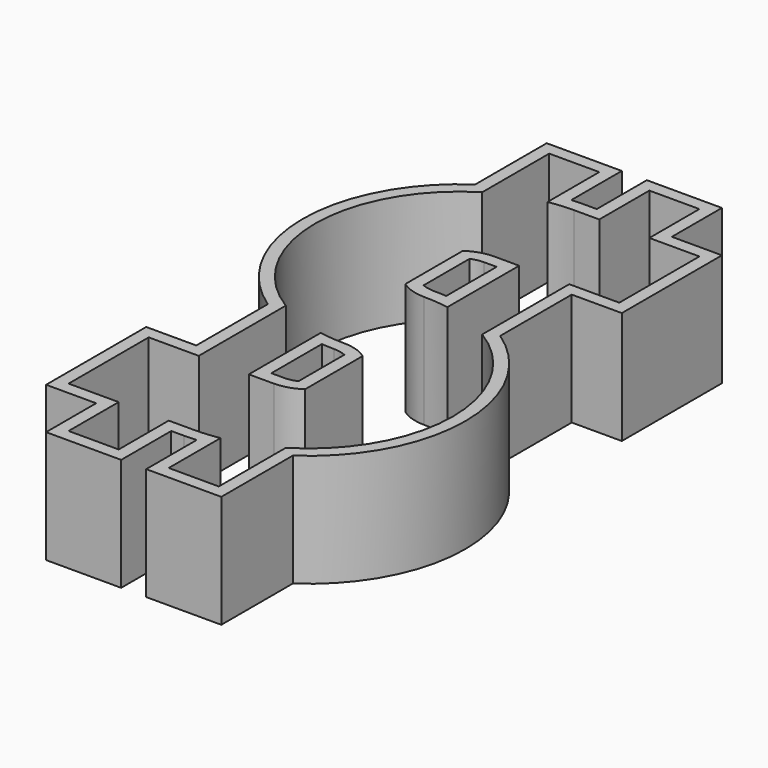
from build123d import *

# Parameters (mm, degrees)
F2_W     = 25.4
F2_H     = 25.4
F4_W     = 15.24
F4_H     = 12.7
F5_DEPTH = 25.4
F6_T     = -2.54
F7_DEPTH = 2.54


with BuildPart() as f3:
    # F3: sweep along a path in F0
    with BuildLine(Plane.XY) as f3_path:
        Line((27.94, 38.1), (0, 38.1))
        ThreePointArc((0, 38.1), (-19.05, 19.05), (0, 0))
        ThreePointArc((0, 0), (19.05, -19.05), (0, -38.1))
        Line((0, -38.1), (-27.94, -38.1))
    # F2 (on offset) → F3 (sweep)
    with BuildSketch(Plane.YZ.offset(27.94)):
        with Locations((38.1, 0)):
            Rectangle(F2_W, F2_H)
    sweep(path=f3_path.line)

    # F4 (on face) → F5 (join)
    with BuildSketch(Plane.XY.offset(12.7)):
        with BuildLine():
            Line((-2.54, 63.5), (-17.78, 63.5))
            Line((-17.78, 63.5), (-17.78, 45.3546402751))
            ThreePointArc((-17.78, 45.3546402751), (-10.5054322267, 49.0116153391), (-2.54, 50.6982369177))
            Line((-2.54, 50.6982369177), (-2.54, 63.5))
        make_face()
        with BuildLine():
            ThreePointArc((-2.54, 50.6982369177), (-10.5054322267, 49.0116153391), (-17.78, 45.3546402751))
            Line((-17.78, 45.3546402751), (-17.78, -7.2546402751))
            ThreePointArc((-17.78, -7.2546402751), (-10.5054322267, -10.9116153391), (-2.54, -12.5982369177))
            Line((-2.54, -12.5982369177), (-2.54, 13.2301288674))
            ThreePointArc((-2.54, 13.2301288674), (-6.35, 19.05), (-2.54, 24.8698711326))
            Line((-2.54, 24.8698711326), (-2.54, 50.6982369177))
        make_face()
        with BuildLine():
            ThreePointArc((-2.54, -12.5982369177), (-10.5054322267, -10.9116153391), (-17.78, -7.2546402751))
            Line((-17.78, -7.2546402751), (-17.78, -25.4))
            Line((-17.78, -25.4), (-2.54, -25.4))
            Line((-2.54, -25.4), (-2.54, -12.5982369177))
        make_face()
        with BuildLine():
            Line((-2.54, 13.2301288674), (-2.54, 24.8698711326))
            ThreePointArc((-2.54, 24.8698711326), (-6.35, 19.05), (-2.54, 13.2301288674))
        make_face()
        with Locations((10.16, 57.15)):
            Rectangle(F4_W, F4_H)
        with Locations((-10.16, -57.15)):
            Rectangle(F4_W, F4_H)
        with BuildLine():
            Line((17.78, 25.4), (2.54, 25.4))
            Line((2.54, 25.4), (2.54, 12.5982369177))
            ThreePointArc((2.54, 12.5982369177), (10.5054322267, 10.9116153391), (17.78, 7.2546402751))
            Line((17.78, 7.2546402751), (17.78, 25.4))
        make_face()
        with BuildLine():
            ThreePointArc((2.54, -24.8698711326), (6.35, -19.05), (2.54, -13.2301288674))
            Line((2.54, -13.2301288674), (2.54, -24.8698711326))
        make_face()
        with BuildLine():
            ThreePointArc((17.78, -45.3546402751), (10.5054322267, -49.0116153391), (2.54, -50.6982369177))
            Line((2.54, -50.6982369177), (2.54, -63.5))
            Line((2.54, -63.5), (17.78, -63.5))
            Line((17.78, -63.5), (17.78, -45.3546402751))
        make_face()
    extrude(amount=-F5_DEPTH)

    # F6
    f6_openings = [f3.faces().sort_by_distance(p)[0] for p in [
        (0, 0, 12.7),
    ]]
    offset(amount=F6_T, openings=f6_openings, kind=Kind.INTERSECTION)

    # F7 (cut): a face of the model
    f7_faces = [f3.faces().sort_by_distance(p)[0] for p in [
        (0, 0, -12.7),
    ]]
    extrude(f7_faces, amount=-F7_DEPTH, mode=Mode.SUBTRACT)


solid = f3.part
